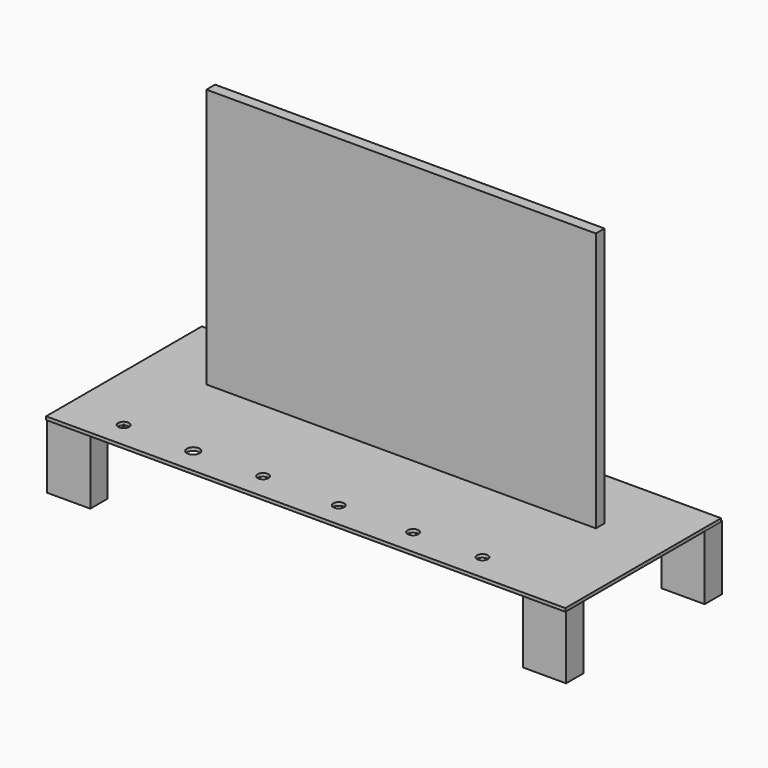
from build123d import *

# Parameters (mm, degrees)
F0_W     = 914.4
F0_H     = 609.6
F1_DEPTH = 25.4
F4_W     = 101.6
F4_H     = 50.8
F5_DEPTH = 152.4
F6_W     = 1219.2
F6_H     = 457.2
F7_DEPTH = 7.62
F8_R     = 12.7
F8_R_2   = 1.5875
F8_R_3   = 14.868698601
F9_DEPTH = 617.2737575347


# Not quite as in the source:
# - the program builds the solid bodies; features that only make, move or delete a surface that nothing else refers to are left out


with BuildPart() as f1:
    # F0 (on Front) → F1 (new body)
    with BuildSketch(Plane.XZ):
        with Locations((410.367934819, 312.4727575347)):
            Rectangle(F0_W, F0_H)
    extrude(amount=F1_DEPTH)


with BuildPart() as f5:
    # F4 (on Top) → F5 (new body)
    with BuildSketch(Plane.XY):
        with Locations((-147.961716485, -278.0494519234)):
            Rectangle(F4_W, F4_H)
    extrude(amount=-F5_DEPTH)


with BuildPart() as f5b:
    # F4 (on Top) → F5, piece 2 (new body)
    with BuildSketch(Plane.XY):
        with Locations((968.5793860435, 129.4654405951)):
            Rectangle(F4_W, F4_H)
    extrude(amount=-F5_DEPTH)


with BuildPart() as f5c:
    # F4 (on Top) → F5, piece 3 (new body)
    with BuildSketch(Plane.XY):
        with Locations((966.5820940018, -274.6879585743)):
            Rectangle(F4_W, F4_H)
    extrude(amount=-F5_DEPTH)


with BuildPart() as f5d:
    # F4 (on Top) → F5, piece 4 (new body)
    with BuildSketch(Plane.XY):
        with Locations((-146.0218621969, 124.194490099)):
            Rectangle(F4_W, F4_H)
    extrude(amount=-F5_DEPTH)


with BuildPart() as f7:
    # F6 (on Top) → F7 (new body)
    with BuildSketch(Plane.XY):
        with Locations((411.9497016907, -78.913833046)):
            Rectangle(F6_W, F6_H)
    extrude(amount=F7_DEPTH)

    # F8 (on Top) → F9 (cut, through all)
    with BuildSketch(Plane.XY):
        with Locations((-65.2297735214, -245.472446084)):
            Circle(F8_R)
        with Locations((-65.2297735214, -245.472446084)):
            Circle(F8_R_2, mode=Mode.SUBTRACT)
        with Locations((99.1470590234, -246.4373856783)):
            Circle(F8_R_3)
        with Locations((261.5713775158, -244.6326613426)):
            Circle(F8_R)
        with Locations((442.0428872108, -248.2420802116)):
            Circle(F8_R)
        with Locations((615.2955293655, -246.4373856783)):
            Circle(F8_R)
        with Locations((776.6676545143, -244.6326613426)):
            Circle(F8_R)
    extrude(amount=F9_DEPTH, mode=Mode.SUBTRACT)


solid = Compound([f1.part, f5.part, f5b.part, f5c.part, f5d.part, f7.part])
